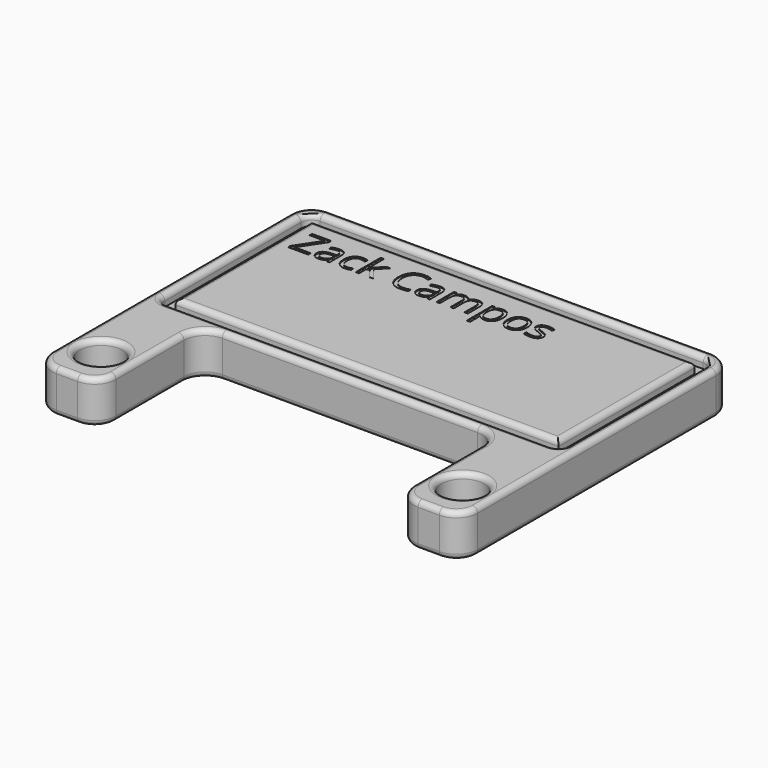
from build123d import *

# Parameters (mm, degrees)
F0_W         = 38.1
F0_H         = 76.2
F1_DEPTH     = 25.4
F2_R         = 12.7
F3_DEPTH     = 25.4
F5_DEPTH     = 6.35
F6_R         = 6.35
F7_R         = 12.7
F8_R         = 3.17499
F9_TEXT_SIZE = 24.4581347538
F10_DEPTH    = 0.508


# Not quite as in the source:
# - a fillet or chamfer is up to 0.001 mm smaller than in the source, because OpenCascade refuses the exact size
# - Text() gives the source's letters only with a copy of the font that has no kerning and outlines rounded to 1/6400 em; it was checked with that copy


with BuildPart() as f1:
    # F0 (on Top) → F1 (new body)
    with BuildSketch(Plane.XY):
        Polygon((0, 127), (0, 0), (38.1, 0), (215.9, 0), (254, 0), (254, 127), align=None)
        with Locations((19.05, -38.1)):
            Rectangle(F0_W, F0_H)
        with Locations((234.95, -38.1)):
            Rectangle(F0_W, F0_H)
    extrude(amount=F1_DEPTH)

    # F2 (on face) → F3 (cut)
    with BuildSketch(Plane.XY.offset(25.4)):
        with Locations((19.05, -50.8)):
            Circle(F2_R)
        with Locations((234.95, -50.8)):
            Circle(F2_R)
    extrude(amount=-F3_DEPTH, mode=Mode.SUBTRACT)

    # F4 (on face) → F5 (cut)
    with BuildSketch(Plane.XY.offset(25.4)):
        Polygon((6.35, 120.65), (6.35, 6.35), (31.75, 6.35), (222.25, 6.35), (247.65, 6.35), (247.65, 120.65), align=None)
        Polygon((31.75, 12.7), (12.7, 12.7), (12.7, 114.3), (241.3, 114.3), (241.3, 12.7), (222.25, 12.7), align=None, mode=Mode.SUBTRACT)
    extrude(amount=-F5_DEPTH, mode=Mode.SUBTRACT)

    # F6
    f6_edges = [f1.edges().sort_by_distance(p)[0] for p in [
        (6.35, 120.65, 22.225),
        (247.65, 120.65, 22.225),
        (247.65, 6.35, 22.225),
        (6.35, 6.35, 22.225),
    ]]
    fillet(f6_edges, radius=F6_R)

    # F7
    f7_edges = [f1.edges().sort_by_distance(p)[0] for p in [
        (254, -76.2, 12.7),
        (215.9, -76.2, 12.7),
        (38.1, -76.2, 12.7),
        (0, -76.2, 12.7),
        (0, 127, 12.7),
        (254, 127, 12.7),
        (38.1, 0, 12.7),
        (215.9, 0, 12.7),
    ]]
    fillet(f7_edges, radius=F7_R)

    # F8 (radius 3.175 in the source; OpenCascade refuses exactly that, so slightly less here)
    f8_edges = [f1.edges().sort_by_distance(p)[0] for p in [
        (12.7, 63.5, 25.4),
        (127, 114.3, 25.4),
        (241.3, 63.5, 25.4),
        (127, 12.7, 25.4),
        (0, 25.4, 25.4),
        (3.719744, 123.280256, 25.4),
        (3.719744, -72.480256, 25.4),
        (127, 127, 25.4),
        (19.05, -76.2, 25.4),
        (250.280256, 123.280256, 25.4),
        (34.380256, -72.480256, 25.4),
        (254, 25.4, 25.4),
        (38.1, -38.1, 25.4),
        (250.280256, -72.480256, 25.4),
        (41.819744, -3.719744, 25.4),
        (234.95, -76.2, 25.4),
        (127, 0, 25.4),
        (219.619744, -72.480256, 25.4),
        (212.180256, -3.719744, 25.4),
        (215.9, -38.1, 25.4),
        (6.35, 63.5, 25.4),
        (8.209872, 118.790128, 25.4),
        (8.209872, 8.209872, 25.4),
        (127, 120.65, 25.4),
        (127, 6.35, 25.4),
        (245.790128, 118.790128, 25.4),
        (245.790128, 8.209872, 25.4),
        (247.65, 63.5, 25.4),
        (6.35, -50.8, 25.4),
        (222.25, -50.8, 25.4),
        (0, 25.4, 0),
        (3.719744, 123.280256, 0),
        (3.719744, -72.480256, 0),
        (127, 127, 0),
        (19.05, -76.2, 0),
        (250.280256, 123.280256, 0),
        (34.380256, -72.480256, 0),
        (254, 25.4, 0),
        (38.1, -38.1, 0),
        (250.280256, -72.480256, 0),
        (41.819744, -3.719744, 0),
        (234.95, -76.2, 0),
        (127, 0, 0),
        (219.619744, -72.480256, 0),
        (212.180256, -3.719744, 0),
        (215.9, -38.1, 0),
        (6.35, -50.8, 0),
        (222.25, -50.8, 0),
    ]]
    fillet(f8_edges, radius=F8_R)

    # F9 (on face) → F10 (cut)
    with BuildSketch(Plane.XY.offset(25.4)):
        with Locations((20.1194752008, 86.2688571215)):
            Text('Zack Campos', F9_TEXT_SIZE, font='Open Sans', text_align=(TextAlign.LEFT, TextAlign.BOTTOM))
    extrude(amount=-F10_DEPTH, mode=Mode.SUBTRACT)


solid = f1.part
